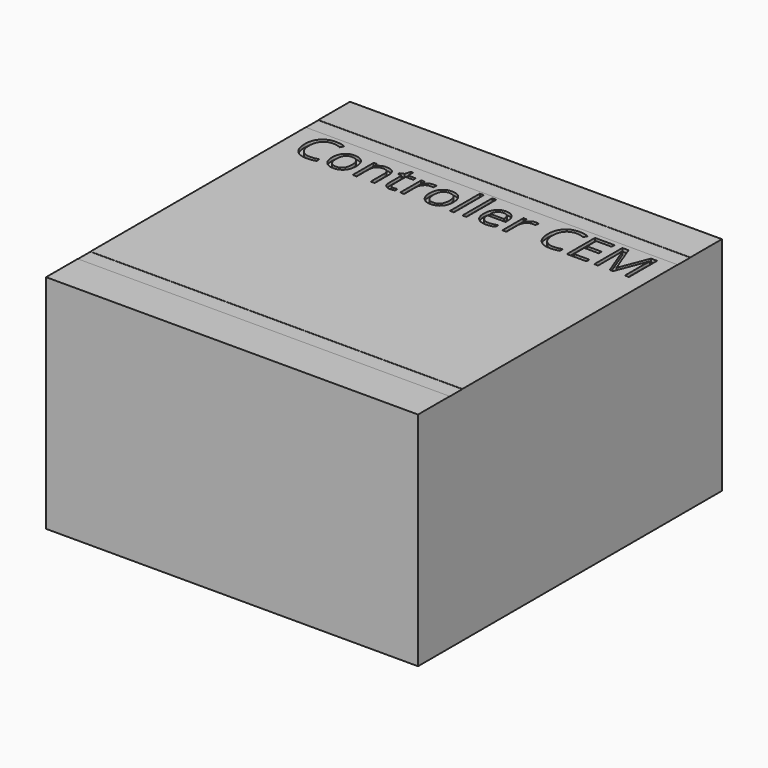
from build123d import *

# Parameters (mm, degrees)
F0_W         = 235
F0_H         = 240
F1_DEPTH     = 140
F2_TEXT_SIZE = 31.0631327744
F3_DEPTH     = 2
F4_W         = 235
F4_H         = 10
F5_DEPTH     = 0.1


# Not quite as in the source:
# - Text() gives the source's letters only with a copy of the font that has no kerning and outlines rounded to 1/6400 em; it was checked with that copy


with BuildPart() as f1:
    # F0 (on Top) → F1 (new body)
    with BuildSketch(Plane.XY):
        Rectangle(F0_W, F0_H)
    extrude(amount=F1_DEPTH)

    # F2 (on face) → F3 (cut)
    with BuildSketch(Plane.XY.offset(140)):
        with Locations((-108.638368547, 59.7543072999)):
            Text('Controller CEM', F2_TEXT_SIZE, font='Open Sans', text_align=(TextAlign.LEFT, TextAlign.BOTTOM))
    extrude(amount=-F3_DEPTH, mode=Mode.SUBTRACT)

    # F4 (on face) → F5 (cut)
    with BuildSketch(Plane.XY.offset(140)):
        with Locations((0, -90)):
            Rectangle(F4_W, F4_H)
        with Locations((0, 90)):
            Rectangle(F4_W, F4_H)
    extrude(amount=-F5_DEPTH, mode=Mode.SUBTRACT)


solid = f1.part
